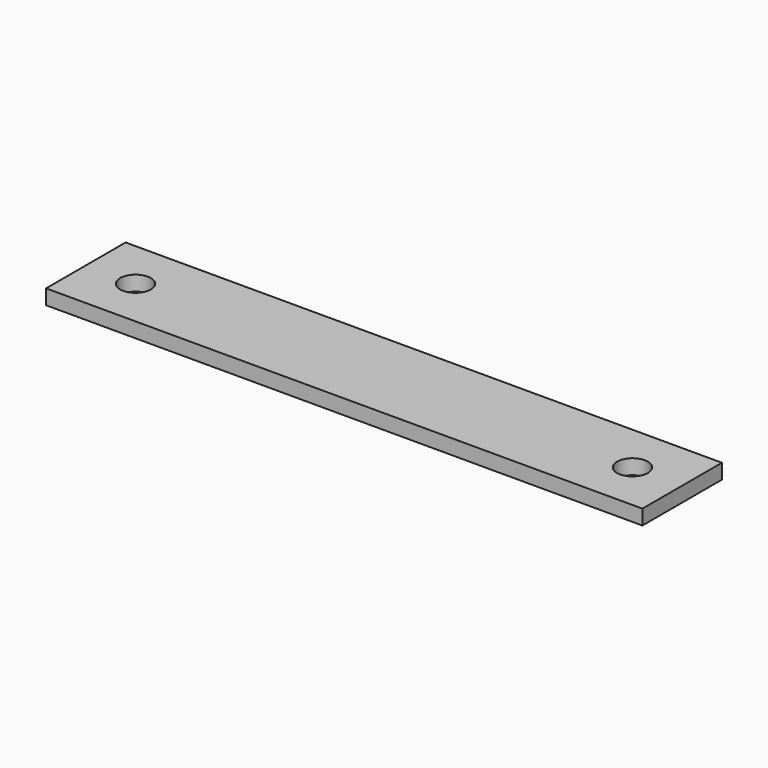
from build123d import *

# Parameters (mm, degrees)
F0_W     = 120
F0_H     = 20
F1_DEPTH = 3
F2_R     = 3.1
F3_DEPTH = 25


# Not quite as in the source:
# - a pattern or mirror of a feature is missing from the dataset's text; its kind, count and spacing are read off the source's solid


with BuildPart() as f1:
    # F0 (on Top) → F1 (new body)
    with BuildSketch(Plane.XY):
        Rectangle(F0_W, F0_H)
    extrude(amount=F1_DEPTH)

    # F2 (on face) → F3 (cut)
    with BuildSketch(Plane.XY.offset(3)):
        with Locations((50, 0)):
            Circle(F2_R)
    f3 = extrude(amount=-F3_DEPTH, mode=Mode.SUBTRACT)

    # F3_copies: F3 across plane
    add(f3.mirror(Plane(origin=(0, 0, 0), x_dir=(0, 0, -1), z_dir=(-1, 0, 0))), mode=Mode.SUBTRACT)


solid = f1.part
